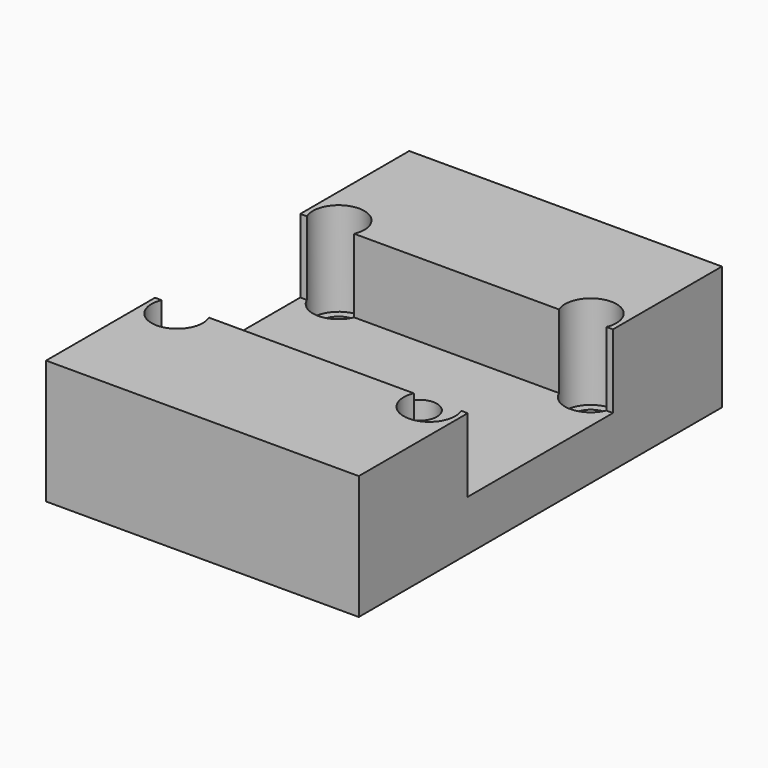
from build123d import *

# Parameters (mm, degrees)
F0_W     = 31
F0_H     = 45
F1_DEPTH = 3
F2_R     = 1.75
F3_DEPTH = 3
F4_DEPTH = 2
F5_DEPTH = 3
F6_DEPTH = 9.3


with BuildPart() as f1:
    # F0 (on Top) → F1 (new body)
    with BuildSketch(Plane.XY):
        with Locations((7.011689, -16.344135)):
            Rectangle(F0_W, F0_H)
    extrude(amount=F1_DEPTH)

    # F2 (on face) → F3 (cut, through all)
    with BuildSketch(Plane.XY.offset(3)):
        with Locations((10.511689, -16.344135)):
            Circle(F2_R)
    extrude(amount=-F3_DEPTH, mode=Mode.SUBTRACT)

    # F2 (on face) → F4 (join)
    with BuildSketch(Plane.XY.offset(3)):
        with BuildLine():
            Line((-7.834052, -25.344135), (-8.488311, -25.344135))
            Line((-8.488311, -25.344135), (-8.488311, -38.844135))
            Line((-8.488311, -38.844135), (22.511689, -38.844135))
            Line((22.511689, -38.844135), (22.511689, -25.344135))
            Line((22.511689, -25.344135), (21.85743, -25.344135))
            ThreePointArc((21.85743, -25.344135), (22.010102, -25.833811), (22.061689, -26.344135))
            ThreePointArc((22.061689, -26.344135), (19.001365, -28.842548), (17.165948, -25.344135))
            Line((17.165948, -25.344135), (-3.14257, -25.344135))
            ThreePointArc((-3.14257, -25.344135), (-2.989898, -25.833811), (-2.938311, -26.344135))
            ThreePointArc((-2.938311, -26.344135), (-5.998635, -28.842548), (-7.834052, -25.344135))
        make_face()
        with BuildLine():
            ThreePointArc((-3.14257, -7.344135), (-5.488311, -8.894135), (-7.834052, -7.344135))
            Line((-7.834052, -7.344135), (-8.488311, -7.344135))
            Line((-8.488311, -7.344135), (-8.488311, -25.344135))
            Line((-8.488311, -25.344135), (-7.834052, -25.344135))
            ThreePointArc((-7.834052, -25.344135), (-5.488311, -23.794135), (-3.14257, -25.344135))
            Line((-3.14257, -25.344135), (17.165948, -25.344135))
            ThreePointArc((17.165948, -25.344135), (19.511689, -23.794135), (21.85743, -25.344135))
            Line((21.85743, -25.344135), (22.511689, -25.344135))
            Line((22.511689, -25.344135), (22.511689, -7.344135))
            Line((22.511689, -7.344135), (21.85743, -7.344135))
            ThreePointArc((21.85743, -7.344135), (19.511689, -8.894135), (17.165948, -7.344135))
            Line((17.165948, -7.344135), (-3.14257, -7.344135))
        make_face()
        with Locations((10.511689, -16.344135)):
            Circle(F2_R, mode=Mode.SUBTRACT)
        with BuildLine():
            Line((-8.488311, -7.344135), (-7.834052, -7.344135))
            ThreePointArc((-7.834052, -7.344135), (-5.998635, -3.845721), (-2.938311, -6.344135))
            ThreePointArc((-2.938311, -6.344135), (-2.989898, -6.854459), (-3.14257, -7.344135))
            Line((-3.14257, -7.344135), (17.165948, -7.344135))
            ThreePointArc((17.165948, -7.344135), (19.001365, -3.845721), (22.061689, -6.344135))
            ThreePointArc((22.061689, -6.344135), (22.010102, -6.854459), (21.85743, -7.344135))
            Line((21.85743, -7.344135), (22.511689, -7.344135))
            Line((22.511689, -7.344135), (22.511689, 6.155865))
            Line((22.511689, 6.155865), (-8.488311, 6.155865))
            Line((-8.488311, 6.155865), (-8.488311, -7.344135))
        make_face()
    extrude(amount=F4_DEPTH)

    # F2 (on face) → F5 (cut, through all)
    with BuildSketch(Plane.XY.offset(3)):
        with BuildLine():
            ThreePointArc((-4.05217, -25.344135), (-5.488311, -24.594135), (-6.924452, -25.344135))
            Line((-6.924452, -25.344135), (-4.05217, -25.344135))
        make_face()
        with BuildLine():
            Line((-4.05217, -25.344135), (-6.924452, -25.344135))
            ThreePointArc((-6.924452, -25.344135), (-6.01236, -28.013827), (-3.738311, -26.344135))
            ThreePointArc((-3.738311, -26.344135), (-3.818618, -25.820086), (-4.05217, -25.344135))
        make_face()
        with BuildLine():
            ThreePointArc((20.94783, -25.344135), (19.511689, -24.594135), (18.075548, -25.344135))
            Line((18.075548, -25.344135), (20.94783, -25.344135))
        make_face()
        with BuildLine():
            Line((20.94783, -25.344135), (18.075548, -25.344135))
            ThreePointArc((18.075548, -25.344135), (18.98764, -28.013827), (21.261689, -26.344135))
            ThreePointArc((21.261689, -26.344135), (21.181382, -25.820086), (20.94783, -25.344135))
        make_face()
        with BuildLine():
            Line((20.94783, -7.344135), (18.075548, -7.344135))
            ThreePointArc((18.075548, -7.344135), (19.511689, -8.094135), (20.94783, -7.344135))
        make_face()
        with BuildLine():
            ThreePointArc((21.261689, -6.344135), (18.98764, -4.674442), (18.075548, -7.344135))
            Line((18.075548, -7.344135), (20.94783, -7.344135))
            ThreePointArc((20.94783, -7.344135), (21.181382, -6.868183), (21.261689, -6.344135))
        make_face()
        with BuildLine():
            Line((-4.05217, -7.344135), (-6.924452, -7.344135))
            ThreePointArc((-6.924452, -7.344135), (-5.488311, -8.094135), (-4.05217, -7.344135))
        make_face()
        with BuildLine():
            ThreePointArc((-4.05217, -7.344135), (-3.818618, -6.868183), (-3.738311, -6.344135))
            ThreePointArc((-3.738311, -6.344135), (-6.01236, -4.674442), (-6.924452, -7.344135))
            Line((-6.924452, -7.344135), (-4.05217, -7.344135))
        make_face()
    extrude(amount=-F5_DEPTH, mode=Mode.SUBTRACT)

    # F2 (on face) → F6 (join)
    with BuildSketch(Plane.XY.offset(3)):
        with BuildLine():
            Line((-8.488311, -7.344135), (-7.834052, -7.344135))
            ThreePointArc((-7.834052, -7.344135), (-5.998635, -3.845721), (-2.938311, -6.344135))
            ThreePointArc((-2.938311, -6.344135), (-2.989898, -6.854459), (-3.14257, -7.344135))
            Line((-3.14257, -7.344135), (17.165948, -7.344135))
            ThreePointArc((17.165948, -7.344135), (19.001365, -3.845721), (22.061689, -6.344135))
            ThreePointArc((22.061689, -6.344135), (22.010102, -6.854459), (21.85743, -7.344135))
            Line((21.85743, -7.344135), (22.511689, -7.344135))
            Line((22.511689, -7.344135), (22.511689, 6.155865))
            Line((22.511689, 6.155865), (-8.488311, 6.155865))
            Line((-8.488311, 6.155865), (-8.488311, -7.344135))
        make_face()
        with BuildLine():
            Line((-7.834052, -25.344135), (-8.488311, -25.344135))
            Line((-8.488311, -25.344135), (-8.488311, -38.844135))
            Line((-8.488311, -38.844135), (22.511689, -38.844135))
            Line((22.511689, -38.844135), (22.511689, -25.344135))
            Line((22.511689, -25.344135), (21.85743, -25.344135))
            ThreePointArc((21.85743, -25.344135), (22.010102, -25.833811), (22.061689, -26.344135))
            ThreePointArc((22.061689, -26.344135), (19.001365, -28.842548), (17.165948, -25.344135))
            Line((17.165948, -25.344135), (-3.14257, -25.344135))
            ThreePointArc((-3.14257, -25.344135), (-2.989898, -25.833811), (-2.938311, -26.344135))
            ThreePointArc((-2.938311, -26.344135), (-5.998635, -28.842548), (-7.834052, -25.344135))
        make_face()
    extrude(amount=F6_DEPTH)


solid = f1.part
